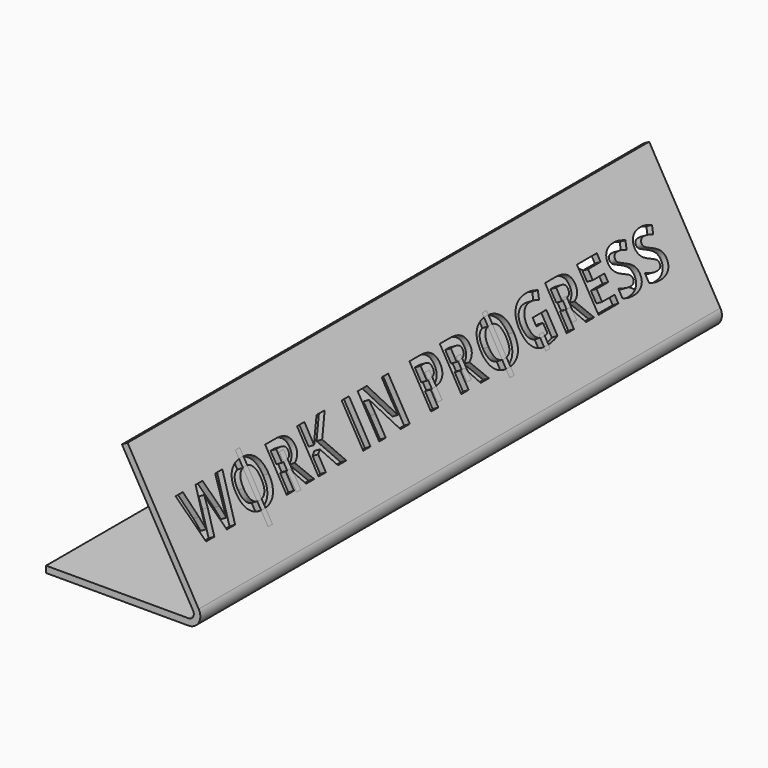
from build123d import *

# Parameters (mm, degrees)
F1_DEPTH     = 120
F2_DEPTH     = 120
F3_R         = 1
F4_R         = 2.2
F6_TEXT_SIZE = 11.1111111111
F7_DEPTH     = 5
F8_W         = 1
F8_H         = 12.0708174072
F8_H_2       = 6.3789670821
F8_H_3       = 4.6990597621
F8_H_4       = 3.9989354555
F8_H_5       = 10.2088246495
F8_H_6       = 3.7902630866
F8_H_7       = 2.5533222361
F9_DEPTH     = 1.2


# Not quite as in the source:
# - Text() gives the source's letters only with a copy of the font that has no kerning and outlines rounded to 1/6400 em; it was checked with that copy


with BuildPart() as f1:
    # F0 (on Front) → F1 (new body)
    with BuildSketch(Plane.XZ):
        Polygon((0, 1.2), (0, 0), (30, 0), (15, 25.9807621135), (13.9607695155, 25.3807621135), (27.9215390309, 1.2), align=None)
    extrude(amount=F1_DEPTH)

    # F0 (on Front) → F2 (join)
    with BuildSketch(Plane.XZ):
        Polygon((0, 1.2), (0, 0), (30, 0), (15, 25.9807621135), (13.9607695155, 25.3807621135), (27.9215390309, 1.2), align=None)
    extrude(amount=F2_DEPTH)

    # F3
    f3_edges = [f1.edges().sort_by_distance(p)[0] for p in [
        (27.921539, -60, 1.2),
    ]]
    fillet(f3_edges, radius=F3_R)

    # F4
    f4_edges = [f1.edges().sort_by_distance(p)[0] for p in [
        (30, -60, 0),
    ]]
    fillet(f4_edges, radius=F4_R)

    # F6 (on face) → F7 (cut)
    with BuildSketch(Plane(origin=(22.5, 0, 12.9903810568), x_dir=(0, 1, 0), z_dir=(0.8660254038, 0, 0.5))):
        with Locations((-115.3457653709, -3.1894882233)):
            Text('WORK IN PROGRESS', F6_TEXT_SIZE, font='Open Sans', font_style=FontStyle.BOLD, text_align=(TextAlign.LEFT, TextAlign.BOTTOM))
    extrude(amount=-F7_DEPTH, mode=Mode.SUBTRACT)

    # F8 (on face) → F9 (join)
    with BuildSketch(Plane(origin=(22.5, 0, 12.9903810568), x_dir=(0, 1, 0), z_dir=(0.8660254038, 0, 0.5))):
        with Locations((-100.1910800934, 0.1829776447)):
            Rectangle(F8_W, F8_H)
        with Locations((-92.2372215867, -0.3825210733)):
            Rectangle(F8_W, F8_H_2)
        with Locations((-59.0912611663, -0.1415209845)):
            Rectangle(F8_W, F8_H_3)
        with Locations((-52.0880655825, -0.0899651786)):
            Rectangle(F8_W, F8_H_4)
        with Locations((-43.8351864815, 0.4468373954)):
            Rectangle(F8_W, F8_H_5)
        with Locations((-27.9597296268, -0.3485286143)):
            Rectangle(F8_W, F8_H_6)
        with Locations((-35.0869978666, -2.6166793541)):
            Rectangle(F8_W, F8_H_7)
    extrude(amount=-F9_DEPTH)


solid = f1.part
